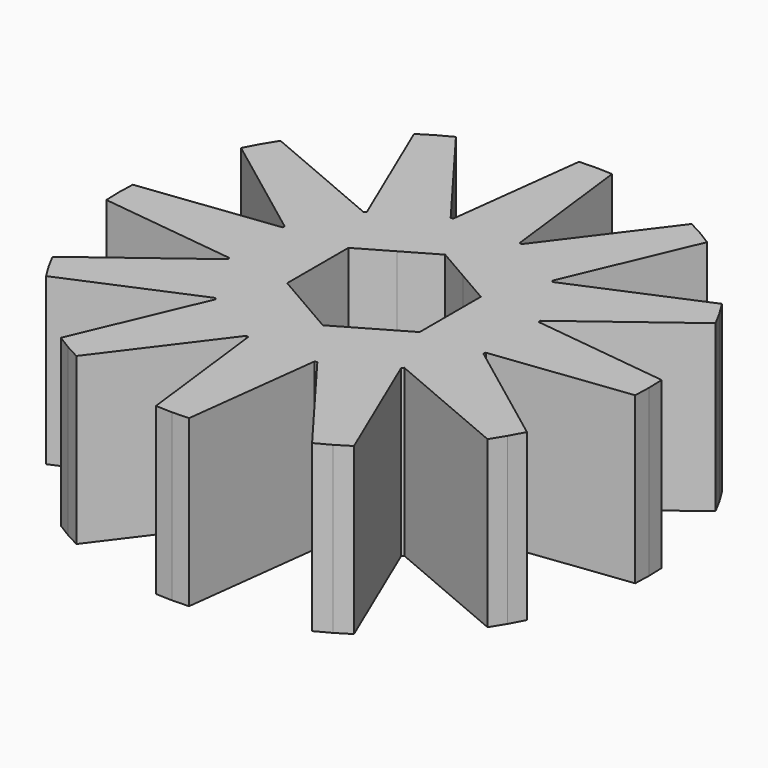
from build123d import *

# Parameters (mm, degrees)
F1_DEPTH = 5


# Not quite as in the source:
# - a feature names something its author has since deleted; it is built from what else it names


with BuildPart() as f1:
    # F0 (on Top) → F1 (new body)
    with BuildSketch(Plane.XY):
        with BuildLine():
            ThreePointArc((-1, 3.8729833462), (0, 4), (1, 3.8729833462))
            Line((1, 3.8729833462), (0.4997557997, 7.984375))
            Line((0.4997557997, 7.984375), (0, 8))
            Line((0, 8), (-0.4997557997, 7.984375))
            Line((-0.4997557997, 7.984375), (-1, 3.8729833462))
        make_face()
        with BuildLine():
            ThreePointArc((4, 0), (3.9681187851, 0.5040171699), (3.8729833462, 1))
            ThreePointArc((3.8729833462, 1), (3.8637033052, 1.0352761804), (3.8541019662, 1.0704662693))
            ThreePointArc((3.8541019662, 1.0704662693), (3.4641016151, 2), (2.8541019662, 2.8025170769))
            ThreePointArc((2.8541019662, 2.8025170769), (2.8284271247, 2.8284271247), (2.8025170769, 2.8541019662))
            ThreePointArc((2.8025170769, 2.8541019662), (2, 3.4641016151), (1.0704662693, 3.8541019662))
            ThreePointArc((1.0704662693, 3.8541019662), (1.0352761804, 3.8637033052), (1, 3.8729833462))
            ThreePointArc((1, 3.8729833462), (0, 4), (-1, 3.8729833462))
            ThreePointArc((-1, 3.8729833462), (-1.0352761804, 3.8637033052), (-1.0704662693, 3.8541019662))
            ThreePointArc((-1.0704662693, 3.8541019662), (-2, 3.4641016151), (-2.8025170769, 2.8541019662))
            ThreePointArc((-2.8025170769, 2.8541019662), (-2.8284271247, 2.8284271247), (-2.8541019662, 2.8025170769))
            ThreePointArc((-2.8541019662, 2.8025170769), (-3.4641016151, 2), (-3.8541019662, 1.0704662693))
            ThreePointArc((-3.8541019662, 1.0704662693), (-3.8637033052, 1.0352761804), (-3.8729833462, 1))
            ThreePointArc((-3.8729833462, 1), (-4, 0), (-3.8729833462, -1))
            ThreePointArc((-3.8729833462, -1), (-3.8637033052, -1.0352761804), (-3.8541019662, -1.0704662693))
            ThreePointArc((-3.8541019662, -1.0704662693), (-3.4641016151, -2), (-2.8541019662, -2.8025170769))
            ThreePointArc((-2.8541019662, -2.8025170769), (-2.8284271247, -2.8284271247), (-2.8025170769, -2.8541019662))
            ThreePointArc((-2.8025170769, -2.8541019662), (-2, -3.4641016151), (-1.0704662693, -3.8541019662))
            ThreePointArc((-1.0704662693, -3.8541019662), (-1.0352761804, -3.8637033052), (-1, -3.8729833462))
            ThreePointArc((-1, -3.8729833462), (0, -4), (1, -3.8729833462))
            ThreePointArc((1, -3.8729833462), (1.0352761804, -3.8637033052), (1.0704662693, -3.8541019662))
            ThreePointArc((1.0704662693, -3.8541019662), (2, -3.4641016151), (2.8025170769, -2.8541019662))
            ThreePointArc((2.8025170769, -2.8541019662), (2.8284271247, -2.8284271247), (2.8541019662, -2.8025170769))
            ThreePointArc((2.8541019662, -2.8025170769), (3.4641016151, -2), (3.8541019662, -1.0704662693))
            ThreePointArc((3.8541019662, -1.0704662693), (3.8637033052, -1.0352761804), (3.8729833462, -1))
            ThreePointArc((3.8729833462, -1), (3.9681187851, -0.5040171699), (4, 0))
        make_face()
        Polygon((2, 1.1547005384), (2, 0), (2, -1.1547005384), (1.0000000433, -1.7320507826), (0, -2.3094010768), (-1.0000000161, -1.7320507983), (-2, -1.1547005384), (-2, 0), (-2, 1.1547005384), (-1.0000000433, 1.7320507826), (0, 2.3094010768), (0.9999999889, 1.732050814), align=None, mode=Mode.SUBTRACT)
        with BuildLine():
            Line((2.8025170769, 2.8541019662), (4.4249887183, 6.6647936835))
            Line((4.4249887183, 6.6647936835), (4, 6.9282032303))
            Line((4, 6.9282032303), (3.5593862817, 7.1645494832))
            Line((3.5593862817, 7.1645494832), (1.0704662693, 3.8541019662))
            ThreePointArc((1.0704662693, 3.8541019662), (2, 3.4641016151), (2.8025170769, 2.8541019662))
        make_face()
        with BuildLine():
            Line((3.8541019662, 1.0704662693), (7.1645494832, 3.5593862817))
            Line((7.1645494832, 3.5593862817), (6.9282032303, 4))
            Line((6.9282032303, 4), (6.6647936835, 4.4249887183))
            Line((6.6647936835, 4.4249887183), (2.8541019662, 2.8025170769))
            ThreePointArc((2.8541019662, 2.8025170769), (3.4641016151, 2), (3.8541019662, 1.0704662693))
        make_face()
        with BuildLine():
            Line((7.984375, -0.4997557997), (8, 0))
            Line((8, 0), (7.984375, 0.4997557997))
            Line((7.984375, 0.4997557997), (3.8729833462, 1))
            ThreePointArc((3.8729833462, 1), (3.9681187851, 0.5040171699), (4, 0))
            ThreePointArc((4, 0), (3.9681187851, -0.5040171699), (3.8729833462, -1))
            Line((3.8729833462, -1), (7.984375, -0.4997557997))
        make_face()
        with BuildLine():
            Line((6.9282032303, -4), (7.1645494832, -3.5593862817))
            Line((7.1645494832, -3.5593862817), (3.8541019662, -1.0704662693))
            ThreePointArc((3.8541019662, -1.0704662693), (3.4641016151, -2), (2.8541019662, -2.8025170769))
            Line((2.8541019662, -2.8025170769), (6.6647936835, -4.4249887183))
            Line((6.6647936835, -4.4249887183), (6.9282032303, -4))
        make_face()
        with BuildLine():
            Line((4, -6.9282032303), (4.4249887183, -6.6647936835))
            Line((4.4249887183, -6.6647936835), (2.8025170769, -2.8541019662))
            ThreePointArc((2.8025170769, -2.8541019662), (2, -3.4641016151), (1.0704662693, -3.8541019662))
            Line((1.0704662693, -3.8541019662), (3.5593862817, -7.1645494832))
            Line((3.5593862817, -7.1645494832), (4, -6.9282032303))
        make_face()
        with BuildLine():
            Line((0.4997557997, -7.984375), (1, -3.8729833462))
            ThreePointArc((1, -3.8729833462), (0, -4), (-1, -3.8729833462))
            Line((-1, -3.8729833462), (-0.4997557997, -7.984375))
            Line((-0.4997557997, -7.984375), (0, -8))
            Line((0, -8), (0.4997557997, -7.984375))
        make_face()
        with BuildLine():
            Line((-3.5593862817, -7.1645494832), (-1.0704662693, -3.8541019662))
            ThreePointArc((-1.0704662693, -3.8541019662), (-2, -3.4641016151), (-2.8025170769, -2.8541019662))
            Line((-2.8025170769, -2.8541019662), (-4.4249887183, -6.6647936835))
            Line((-4.4249887183, -6.6647936835), (-4, -6.9282032303))
            Line((-4, -6.9282032303), (-3.5593862817, -7.1645494832))
        make_face()
        with BuildLine():
            Line((-6.6647936835, -4.4249887183), (-2.8541019662, -2.8025170769))
            ThreePointArc((-2.8541019662, -2.8025170769), (-3.4641016151, -2), (-3.8541019662, -1.0704662693))
            Line((-3.8541019662, -1.0704662693), (-7.1645494832, -3.5593862817))
            Line((-7.1645494832, -3.5593862817), (-6.9282032303, -4))
            Line((-6.9282032303, -4), (-6.6647936835, -4.4249887183))
        make_face()
        with BuildLine():
            ThreePointArc((-3.8729833462, -1), (-4, 0), (-3.8729833462, 1))
            Line((-3.8729833462, 1), (-7.984375, 0.4997557997))
            Line((-7.984375, 0.4997557997), (-8, 0))
            Line((-8, 0), (-7.984375, -0.4997557997))
            Line((-7.984375, -0.4997557997), (-3.8729833462, -1))
        make_face()
        with BuildLine():
            ThreePointArc((-3.8541019662, 1.0704662693), (-3.4641016151, 2), (-2.8541019662, 2.8025170769))
            Line((-2.8541019662, 2.8025170769), (-6.6647936835, 4.4249887183))
            Line((-6.6647936835, 4.4249887183), (-6.9282032303, 4))
            Line((-6.9282032303, 4), (-7.1645494832, 3.5593862817))
            Line((-7.1645494832, 3.5593862817), (-3.8541019662, 1.0704662693))
        make_face()
        with BuildLine():
            ThreePointArc((-2.8025170769, 2.8541019662), (-2, 3.4641016151), (-1.0704662693, 3.8541019662))
            Line((-1.0704662693, 3.8541019662), (-3.5593862817, 7.1645494832))
            Line((-3.5593862817, 7.1645494832), (-4, 6.9282032303))
            Line((-4, 6.9282032303), (-4.4249887183, 6.6647936835))
            Line((-4.4249887183, 6.6647936835), (-2.8025170769, 2.8541019662))
        make_face()
    extrude(amount=F1_DEPTH)


solid = f1.part
